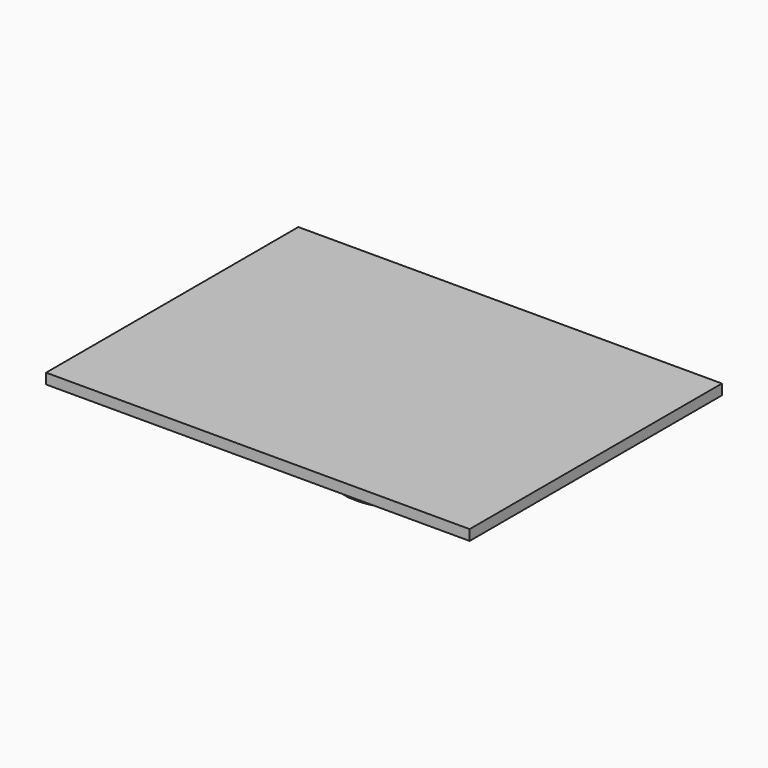
from build123d import *

# Parameters (mm, degrees)
F0_TEXT_SIZE = 58.2400295469
F1_DEPTH     = 5
F3_START     = 4
F2_W         = 202.7765512466
F2_H         = 150.9604156017
F3_DEPTH     = 5


# Not quite as in the source:
# - Text() gives the source's letters only with a copy of the font that has no kerning and outlines rounded to 1/6400 em; it was checked with that copy


with BuildPart() as f1:
    # F0 (on Top) → F1 (new body)
    with BuildSketch(Plane.XY):
        with BuildLine():
            add(Edge.make_bspline(
                [(-26.7019018583, -4.9264831727), (-22.3475496492, -0.6722310144), (-22.3475496492, 7.6542732099)],
                knots=[0, 0, 0, 1, 1, 1], degree=2))
            add(Edge.make_bspline(
                [(-22.3475496492, 7.6542732099), (-22.3475496492, 15.7896773372), (-26.4289017198, 19.9119794286)],
                knots=[0, 0, 0, 1, 1, 1], degree=2))
            add(Edge.make_bspline(
                [(-26.4289017198, 19.9119794286), (-30.5102537904, 24.03428152), (-38.5637578761, 24.03428152)],
                knots=[0, 0, 0, 1, 1, 1], degree=2))
            Line((-38.5637578761, 24.03428152), (-45.5889614402, 24.03428152))
            Line((-45.5889614402, 24.03428152), (-45.5889614402, -9.180735331))
            Line((-45.5889614402, -9.180735331), (-39.7012584532, -9.180735331))
            add(Edge.make_bspline(
                [(-39.7012584532, -9.180735331), (-31.0562540674, -9.180735331), (-26.7019018583, -4.9264831727)],
                knots=[0, 0, 0, 1, 1, 1], degree=2))
        make_face()
        with BuildLine():
            add(Edge.make_bspline(
                [(67.8061960886, -93.3876280518), (66.0134951791, -94.9209788297), (66.0134951791, -97.7965802886)],
                knots=[0, 0, 0, 1, 1, 1], degree=2))
            add(Edge.make_bspline(
                [(66.0134951791, -97.7965802886), (66.0134951791, -100.326381572), (68.1474462617, -101.6367822368)],
                knots=[0, 0, 0, 1, 1, 1], degree=2))
            add(Edge.make_bspline(
                [(68.1474462617, -101.6367822368), (70.2813973443, -102.9471829016), (74.2580993618, -102.9471829016)],
                knots=[0, 0, 0, 1, 1, 1], degree=2))
            add(Edge.make_bspline(
                [(74.2580993618, -102.9471829016), (80.2004023766, -102.9471829016), (83.0578038262, -101.1681319991)],
                knots=[0, 0, 0, 1, 1, 1], degree=2))
            add(Edge.make_bspline(
                [(83.0578038262, -101.1681319991), (85.9152052758, -99.3890810965), (85.9152052758, -96.3496795545)],
                knots=[0, 0, 0, 1, 1, 1], degree=2))
            add(Edge.make_bspline(
                [(85.9152052758, -96.3496795545), (85.9152052758, -93.8198782711), (84.3545544841, -92.8370777725)],
                knots=[0, 0, 0, 1, 1, 1], degree=2))
            add(Edge.make_bspline(
                [(84.3545544841, -92.8370777725), (82.7939036923, -91.8542772738), (78.4714014994, -91.8542772738)],
                knots=[0, 0, 0, 1, 1, 1], degree=2))
            Line((78.4714014994, -91.8542772738), (72.8111986278, -91.8542772738))
            add(Edge.make_bspline(
                [(72.8111986278, -91.8542772738), (69.5988969981, -91.8542772738), (67.8061960886, -93.3876280518)],
                knots=[0, 0, 0, 1, 1, 1], degree=2))
        make_face()
        with BuildLine():
            add(Edge.make_bspline(
                [(70.3632973859, -66.0603141878), (68.5705964764, -67.848465095), (68.5705964764, -71.3792668862)],
                knots=[0, 0, 0, 1, 1, 1], degree=2))
            add(Edge.make_bspline(
                [(68.5705964764, -71.3792668862), (68.5705964764, -74.6461685436), (70.4178974136, -76.3251193954)],
                knots=[0, 0, 0, 1, 1, 1], degree=2))
            add(Edge.make_bspline(
                [(70.4178974136, -76.3251193954), (72.2651983508, -78.0040702472), (75.5685000266, -78.0040702472)],
                knots=[0, 0, 0, 1, 1, 1], degree=2))
            add(Edge.make_bspline(
                [(75.5685000266, -78.0040702472), (82.4754035307, -78.0040702472), (82.4754035307, -71.2882668401)],
                knots=[0, 0, 0, 1, 1, 1], degree=2))
            add(Edge.make_bspline(
                [(82.4754035307, -71.2882668401), (82.4754035307, -64.2721632806), (75.4865999851, -64.2721632806)],
                knots=[0, 0, 0, 1, 1, 1], degree=2))
            add(Edge.make_bspline(
                [(75.4865999851, -64.2721632806), (72.1559982954, -64.2721632806), (70.3632973859, -66.0603141878)],
                knots=[0, 0, 0, 1, 1, 1], degree=2))
        make_face()
        with BuildLine():
            add(Edge.make_bspline(
                [(-4.5024405958, -8.693885084), (-2.955439811, -10.0270357604), (-0.1708383982, -10.0270357604)],
                knots=[0, 0, 0, 1, 1, 1], degree=2))
            add(Edge.make_bspline(
                [(-0.1708383982, -10.0270357604), (4.2426638409, -10.0270357604), (6.7588151174, -7.6109845346)],
                knots=[0, 0, 0, 1, 1, 1], degree=2))
            add(Edge.make_bspline(
                [(6.7588151174, -7.6109845346), (9.2749663939, -5.1949333089), (9.2749663939, -0.8451311021)],
                knots=[0, 0, 0, 1, 1, 1], degree=2))
            Line((9.2749663939, -0.8451311021), (9.2749663939, 1.9667703244))
            Line((9.2749663939, 1.9667703244), (4.5520639978, 1.7756702275))
            add(Edge.make_bspline(
                [(4.5520639978, 1.7756702275), (-1.0808388599, 1.5754701259), (-3.5651401203, 0.0239193388)],
                knots=[0, 0, 0, 1, 1, 1], degree=2))
            add(Edge.make_bspline(
                [(-3.5651401203, 0.0239193388), (-6.0494413806, -1.5276314484), (-6.0494413806, -4.7945331058)],
                knots=[0, 0, 0, 1, 1, 1], degree=2))
            add(Edge.make_bspline(
                [(-6.0494413806, -4.7945331058), (-6.0494413806, -7.3607344077), (-4.5024405958, -8.693885084)],
                knots=[0, 0, 0, 1, 1, 1], degree=2))
        make_face()
        with BuildLine():
            add(Edge.make_bspline(
                [(91.7710582467, 12.0495754398), (89.7827072379, 14.4246766447), (86.0790053589, 14.4246766447)],
                knots=[0, 0, 0, 1, 1, 1], degree=2))
            add(Edge.make_bspline(
                [(86.0790053589, 14.4246766447), (82.3298034569, 14.4246766447), (80.0957523235, 11.9813254051)],
                knots=[0, 0, 0, 1, 1, 1], degree=2))
            add(Edge.make_bspline(
                [(80.0957523235, 11.9813254051), (77.8617011901, 9.5379741655), (77.4613009869, 5.2154719726)],
                knots=[0, 0, 0, 1, 1, 1], degree=2))
            Line((77.4613009869, 5.2154719726), (93.7594092555, 5.2154719726))
            add(Edge.make_bspline(
                [(93.7594092555, 5.2154719726), (93.7594092555, 9.6744742348), (91.7710582467, 12.0495754398)],
                knots=[0, 0, 0, 1, 1, 1], degree=2))
        make_face()
        with Locations((-25.8692514358, -92.564077634)):
            Text('King', F0_TEXT_SIZE, font='Open Sans', text_align=(TextAlign.LEFT, TextAlign.BOTTOM))
        with Locations((-56.135866791, -13.3576374501)):
            Text('Daniel', F0_TEXT_SIZE, font='Open Sans', text_align=(TextAlign.LEFT, TextAlign.BOTTOM))
    extrude(amount=F1_DEPTH)


with BuildPart() as f3:
    # F2 (on Top) → F3 (new body)
    with BuildSketch(Plane.XY.offset(F3_START)):
        with Locations((31.6200852394, -36.1080989242)):
            Rectangle(F2_W, F2_H)
    extrude(amount=F3_DEPTH)


solid = Compound([f1.part, f3.part])
